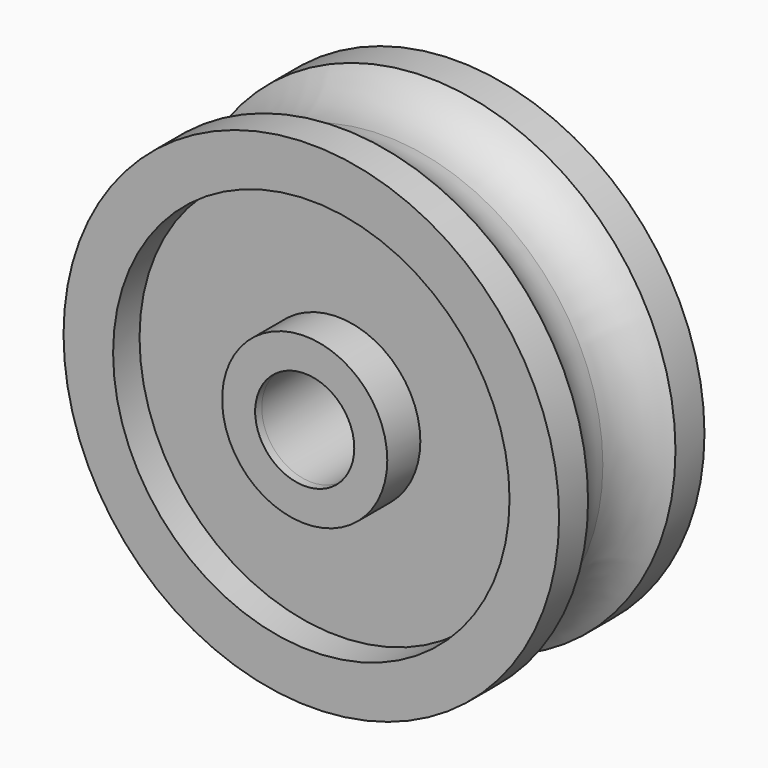
from build123d import *
from build123d import SkipClean  # not in build123d's __all__

# Parameters (mm, degrees)
F2_R     = 5
F2_R_2   = 3
F3_DEPTH = 0.5
F2_R_3   = 12
F4_DEPTH = 2
F5_DEPTH = 25


with BuildPart() as f1:
    # F0 (on Top) → F1 (revolve)
    with BuildSketch(Plane.XY):
        with BuildLine():
            Line((0, -5.5), (0, 0))
            Line((0, 0), (-13.25, 0))
            ThreePointArc((-13.25, 0), (-13.7144660941, -1.8708286934), (-15, -3.3071891388))
            Line((-15, -3.3071891388), (-15, -5.5))
            Line((-15, -5.5), (0, -5.5))
        make_face()
    revolve(axis=Axis((0, -2.75, 0), (0, -1, 0)))

    # F2 (on face) → F3 (join)
    with BuildSketch(Plane.XZ.offset(5.5)):
        Circle(F2_R)
        Circle(F2_R_2, mode=Mode.SUBTRACT)
    extrude(amount=F3_DEPTH)

    # F2 (on face) → F4 (cut)
    with BuildSketch(Plane.XZ.offset(5.5)):
        Circle(F2_R_3)
        Circle(F2_R, mode=Mode.SUBTRACT)
    extrude(amount=-F4_DEPTH, mode=Mode.SUBTRACT)

    # F5 (cut): a face of the model
    f5_faces = [f1.faces().sort_by_distance(p)[0] for p in [
        (0, -5.5, 0),
    ]]
    extrude(f5_faces, amount=-F5_DEPTH, mode=Mode.SUBTRACT)

    # F6: F1 across plane


with BuildPart() as f1_1:
    add(f1.part, clean=False)
    with SkipClean():  # cleaning this boolean's faces spoils the solid; the shape is the same uncleaned
        add(f1.part.mirror(Plane.XZ), clean=False)


solid = f1_1.part
